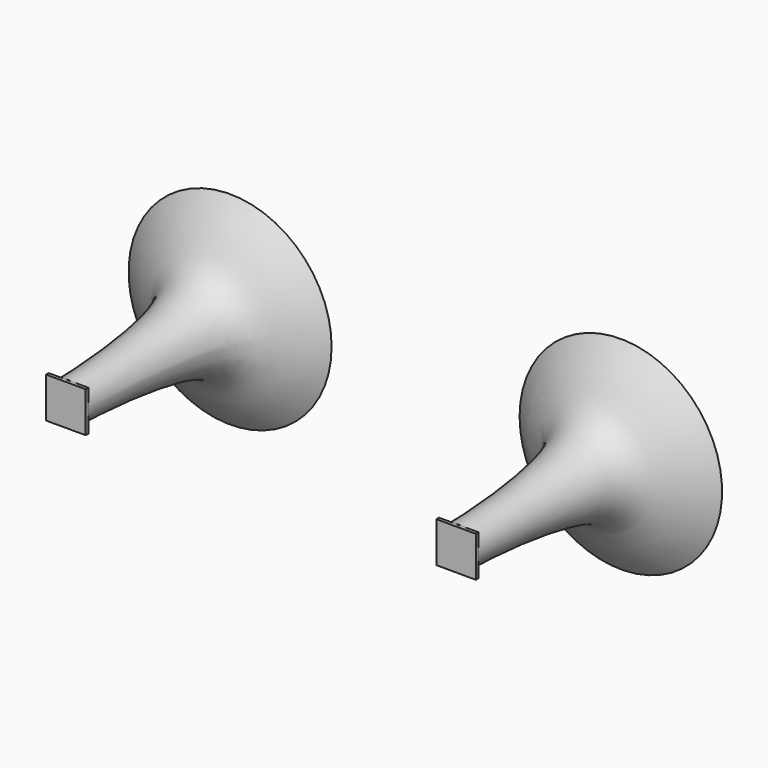
from build123d import *

# Parameters (mm, degrees)
F0_W          = 6.35
F0_H          = 1.0640472173
F3_DEPTH      = 6.25564
F3_DEPTH_BACK = 6.72088
F5_R          = 12.7
F5_2_R        = 12.7


# Not quite as in the source:
# - a feature of the source that left no trace in its solid (it failed there, or was rolled back) is left out


with BuildPart() as f1:
    # F0 (on Top) → F1 (revolve)
    with BuildSketch(Plane.XY):
        with BuildLine():
            add(Edge.make_bspline(
                [(-29.4706169434, 78.933593278), (-40.0197984199, 69.9824278464), (-53.8529486844, 71.986483099), (-55.6433195412, 20.8469636522), (-55.6433195412, 14.2199778929)],
                knots=[0, 0, 0, 0, 0.4242982639, 1, 1, 1, 1], degree=3))
            Line((-29.4706169434, 78.933593278), (-55.6433195412, 78.933593278))
            Line((-55.6433195412, 78.933593278), (-55.6433195412, 14.2199778929))
        make_face()
    revolve(axis=Axis((-61.9933195412, 46.5767855855, 0), (0, 1, 0)))

    # F5#2
    f5_2_edges = [f1.edges().sort_by_distance(p)[0] for p in [
        (-68.34332, 78.933593, 0),
    ]]
    fillet(f5_2_edges, radius=F5_2_R)


with BuildPart() as f3:
    # F0 (on Top) → F3 (new body, two sides)
    with BuildSketch(Plane.XY) as f3_sk:
        with Locations((-58.8183195412, 13.6879542842)):
            Rectangle(F0_W, F0_H)
        with Locations((-65.1683195412, 13.6879542842)):
            Rectangle(F0_W, F0_H)
    extrude(amount=F3_DEPTH)
    extrude(f3_sk.sketch, amount=-F3_DEPTH_BACK)


with BuildPart() as f3b:
    # F0 (on Top) → F3, piece 2 (new body, two sides)
    with BuildSketch(Plane.XY) as f3_2_sk:
        Polygon((63.1731412094, 12.9742378882), (63.1762303644, 14.0382806213), (56.8262571254, 14.0567160194), (56.8231679704, 12.9926732863), align=None)
        Polygon((69.5262036034, 14.0198452232), (63.1762303644, 14.0382806213), (63.1731412094, 12.9742378882), (69.5231144484, 12.9558024901), align=None)
    extrude(amount=F3_DEPTH)
    extrude(f3_2_sk.sketch, amount=-F3_DEPTH_BACK)


with BuildPart() as f4:
    # F0 (on Top) → F4 (revolve)
    with BuildSketch(Plane.XY):
        with BuildLine():
            add(Edge.make_bspline(
                [(30.8415421924, 78.8460435923), (41.3646920775, 69.8642893703), (55.2036022425, 71.8281756051), (56.845496672, 20.6836738504), (56.8262571254, 14.0567160194)],
                knots=[0, 0, 0, 0, 0.4242982639, 1, 1, 1, 1], degree=3))
            Line((56.8262571254, 14.0567160194), (57.0141344898, 78.77005868))
            Line((57.0141344898, 78.77005868), (30.8415421924, 78.8460435923))
        make_face()
    revolve(axis=Axis((63.2701690466, 46.3949519516, 0), (0.0029032123, 0.9999957857, 0)))

    # F5
    f5_edges = [f4.edges().sort_by_distance(p)[0] for p in [
        (69.714081, 78.733188, 0),
    ]]
    fillet(f5_edges, radius=F5_R)


solid = Compound([f1.part, f3.part, f3b.part, f4.part])
